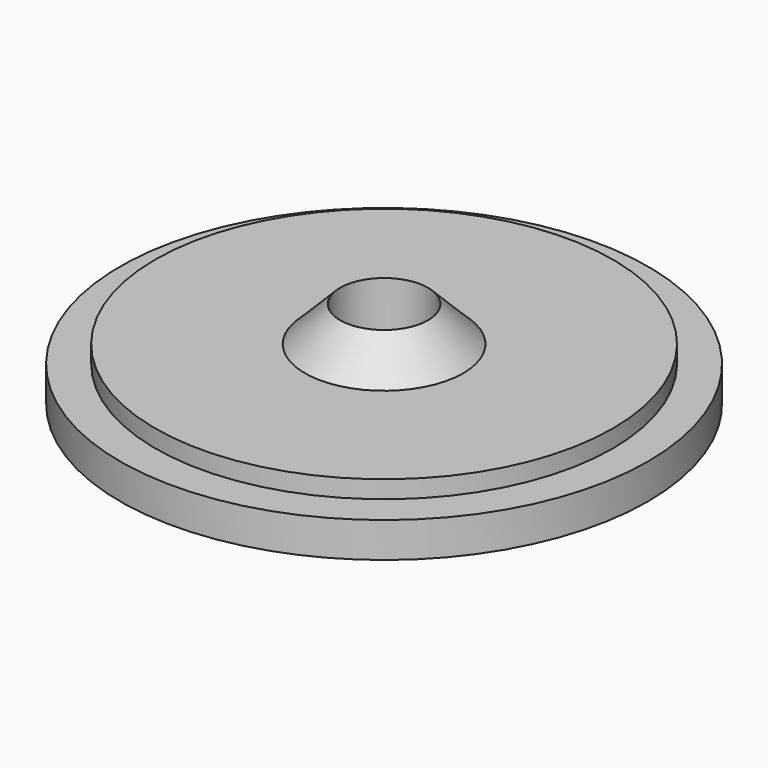
from build123d import *

# Parameters (mm, degrees)
F0_R     = 15
F0_R_2   = 2.5
F1_DEPTH = 2
F2_R     = 13
F2_R_2   = 2.5
F3_DEPTH = 1
F4_R     = 4.5
F4_R_2   = 2.5
F5_DEPTH = 2
F6_SIZE2 = 1.99999
F6_SIZE  = 1.99999


# Not quite as in the source:
# - a fillet or chamfer is up to 0.001 mm smaller than in the source, because OpenCascade refuses the exact size


with BuildPart() as f1:
    # F0 (on Top) → F1 (new body)
    with BuildSketch(Plane.XY):
        Circle(F0_R)
        Circle(F0_R_2, mode=Mode.SUBTRACT)
    extrude(amount=F1_DEPTH)

    # F2 (on face) → F3 (join)
    with BuildSketch(Plane.XY.offset(2)):
        Circle(F2_R)
        Circle(F2_R_2, mode=Mode.SUBTRACT)
    extrude(amount=F3_DEPTH)

    # F4 (on face) → F5 (join)
    with BuildSketch(Plane.XY.offset(3)):
        Circle(F4_R)
        Circle(F4_R_2, mode=Mode.SUBTRACT)
    extrude(amount=F5_DEPTH)

    # F6 (size 2 and 2 in the source; OpenCascade refuses exactly that, so slightly less here)
    f6_edges = [f1.edges().sort_by_distance(p)[0] for p in [
        (-4.5, 0, 5),
    ]]
    chamfer(f6_edges, length=F6_SIZE, length2=F6_SIZE2)


solid = f1.part
